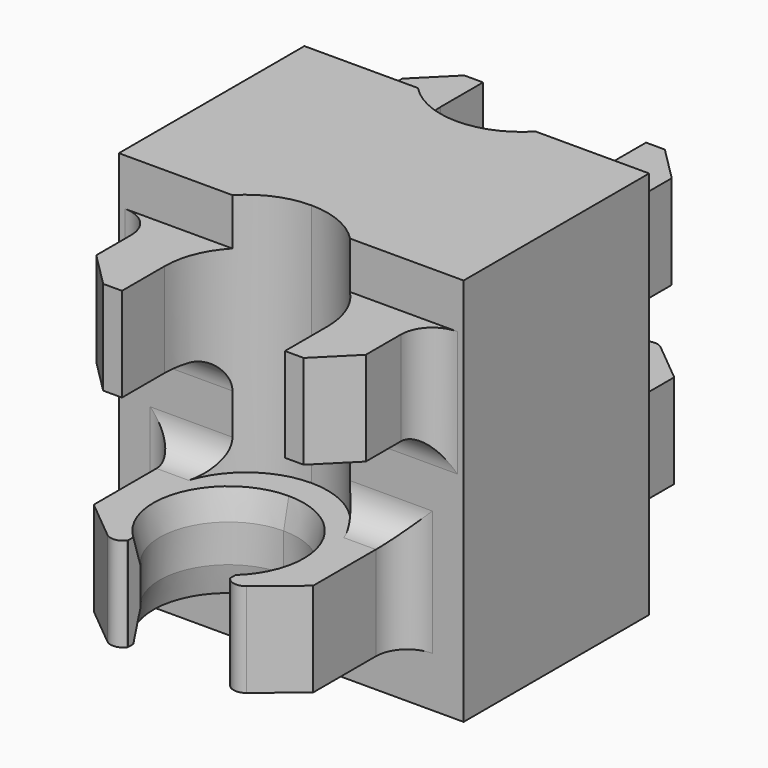
from build123d import *

# Parameters (mm, degrees)
F1_DEPTH  = 12.4
F2_W      = 4.8141676475
F2_H      = 3.3
F2_H_2    = 1.6
F2_H_3    = 1.5
F3_DEPTH  = 25
F5_DEPTH  = 7.8
F6_DEPTH  = 0.8
F7_SIZE   = 1.1
F8_R      = 0.4
F9_R      = 1
F10_SIZE2 = 0.2
F10_SIZE  = 0.9


# Not quite as in the source:
# - a feature of the source that left no trace in its solid (it failed there, or was rolled back) is left out


with BuildPart() as f1:
    # F0 (on Top) → F1 (new body)
    with BuildSketch(Plane.XY):
        with BuildLine():
            ThreePointArc((0, -2.2), (-2.0110712703, -0.8919598342), (-1.6307225426, 1.476734231))
            Line((-1.6307225426, 1.476734231), (-1.6307225426, 1.976734231))
            Line((-1.6307225426, 1.976734231), (-1.9090909091, 2.3141676475))
            Line((-1.9090909091, 2.3141676475), (-3.5, 1.0017346067))
            Line((-3.5, 1.0017346067), (-3.5, -2.5))
            Line((-3.5, -2.5), (-5.5, -2.5))
            Line((-5.5, -2.5), (-5.5, -6.2))
            Line((-5.5, -6.2), (0, -6.2))
            Line((0, -6.2), (0, -2.2))
        make_face()
    extrude(amount=F1_DEPTH)

    # F2 (on face) → F3 (cut)
    with BuildSketch(Plane(origin=(-3.5, 0, 0), x_dir=(0, -1, 0), z_dir=(-1, 0, 0))):
        with Locations((0.0929161762, 6.25)):
            Rectangle(F2_W, F2_H)
        with Locations((0.0929161762, 0.8)):
            Rectangle(F2_W, F2_H_2)
        with Locations((0.0929161762, 11.65)):
            Rectangle(F2_W, F2_H_3)
    extrude(amount=-F3_DEPTH, mode=Mode.SUBTRACT)

    # F4 (on face) → F5 (cut, through all)
    with BuildSketch(Plane.XY.offset(12.4)):
        with BuildLine():
            Line((-2.6, 1.0017346067), (-2.6, -0.7))
            ThreePointArc((-2.6, -0.7), (-1.8384776311, -2.5384776311), (0, -3.3))
            Line((0, -3.3), (0, -2.2))
            ThreePointArc((0, -2.2), (-2.0110712703, -0.8919598342), (-1.6307225426, 1.476734231))
            Line((-1.6307225426, 1.476734231), (-1.6307225426, 1.976734231))
            Line((-1.6307225426, 1.976734231), (-1.9090909091, 2.3141676475))
            Line((-1.9090909091, 2.3141676475), (-3.5, 1.0017346067))
            Line((-3.5, 1.0017346067), (-2.6, 1.0017346067))
        make_face()
    extrude(amount=-F5_DEPTH, mode=Mode.SUBTRACT)

    # F6 (add): a face of the model
    f6_faces = [f1.faces().sort_by_distance(p)[0] for p in [
        (-3.5, -0.7491326967, 9.4),
    ]]
    extrude(f6_faces, amount=F6_DEPTH)

    # F7
    f7_edges = [f1.edges().sort_by_distance(p)[0] for p in [
        (-4.3, 1.001735, 9.4),
    ]]
    chamfer(f7_edges, length=F7_SIZE)

    # F8
    f8_edges = [f1.edges().sort_by_distance(p)[0] for p in [
        (-1.909091, 2.314168, 3.1),
    ]]
    fillet(f8_edges, radius=F8_R)

    # F9
    f9_edges = [f1.edges().sort_by_distance(p)[0] for p in [
        (-3.5, -2.5, 3.1),
        (-2.688083, -2.5, 4.6),
        (-3.088083, -2.5, 7.9),
        (-4.3, -2.5, 9.4),
    ]]
    fillet(f9_edges, radius=F9_R)

    # F10
    f10_edges = [f1.edges().sort_by_distance(p)[0] for p in [
        (-2.011071, -0.89196, 1.6),
        (-2.011071, -0.89196, 4.6),
    ]]
    f10_side = f1.faces().sort_by_distance((-2.011071, -0.89196, 3.1))[0]
    chamfer(f10_edges, length=F10_SIZE, length2=F10_SIZE2, reference=f10_side)

    # F11: F1 across face


with BuildPart() as f1_1:
    add(f1.part)
    add(f1.part.mirror(Plane(origin=(0, -4.5388751239, 5.7890981169), x_dir=(0, 1, 0), z_dir=(1, 0, 0))))

    # F12: F1 across face


with BuildPart() as f1_2:
    add(f1_1.part)
    add(f1_1.part.mirror(Plane(origin=(0, -6.2, 6.2), x_dir=(1, 0, 0), z_dir=(0, -1, 0))))


solid = f1_2.part
